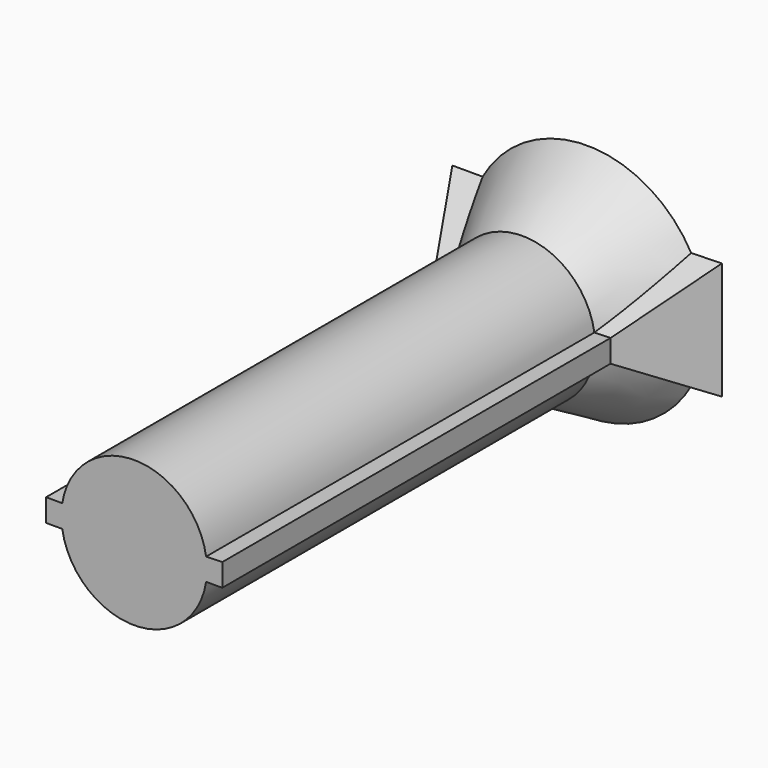
from build123d import *

# Parameters (mm, degrees)
F1_DEPTH               = 150
F2_DEPTH               = 25
DRAFT_F2_DRAFTED_ANGLE = -30


# Not quite as in the source:
# - an extrude with a draft is written as a straight extrude whose walls are then drafted


with BuildPart() as f1:
    # F0 (on Front) → F1 (new body)
    with BuildSketch(Plane.XZ):
        with BuildLine():
            ThreePointArc((22.2314160966, -3.4556680013), (22.4296056885, -1.7411981749), (22.4957987085, -0.0165810045))
            ThreePointArc((22.4957987085, -0.0165810045), (22.4300515903, 1.7022260351), (22.2331944739, 3.4109880427))
            ThreePointArc((22.2331944739, 3.4109880427), (0.0324511096, 22.4833891422), (-22.2303120623, 3.4834189955))
            ThreePointArc((-22.2303120623, 3.4834189955), (-22.5042012915, -0.0165810045), (-22.2303120623, -3.5165810045))
            ThreePointArc((-22.2303120623, -3.5165810045), (0.0266239001, -22.5165598891), (22.2314160966, -3.4556680013))
        make_face()
        with BuildLine():
            ThreePointArc((-22.2303120623, -3.5165810045), (-22.5042012915, -0.0165810045), (-22.2303120623, 3.4834189955))
            Line((-22.2303120623, 3.4834189955), (-27.2303120623, 3.4834189955))
            Line((-27.2303120623, 3.4834189955), (-27.2303120623, -3.5165810045))
            Line((-27.2303120623, -3.5165810045), (-22.2303120623, -3.5165810045))
        make_face()
        with BuildLine():
            ThreePointArc((22.2331944739, 3.4109880427), (22.4300515903, 1.7022260351), (22.4957987085, -0.0165810045))
            ThreePointArc((22.4957987085, -0.0165810045), (22.4296056885, -1.7411981749), (22.2314160966, -3.4556680013))
            Line((22.2314160966, -3.4556680013), (27.2314160966, -3.4556680013))
            Line((27.2314160966, -3.4556680013), (27.2314160966, 3.5443319987))
            Line((27.2314160966, 3.5443319987), (22.2331944739, 3.4109880427))
        make_face()
    extrude(amount=F1_DEPTH)


with BuildPart() as f2_drafted:
    # F2 (new): a face of the model
    f2_faces = [f1.part.faces().sort_by_distance(p)[0] for p in [
        (-0.0079243698, 0, -0.0160022595),
    ]]
    extrude(f2_faces, amount=F2_DEPTH)

    # draft_F2_drafted
    draft_f2_drafted_walls = [f2_drafted.faces().sort_by_distance(p)[0] for p in [
        (-24.7303120623, 16.6666666667, 3.4834189955),
        (-27.2303120623, 16.6666666667, -0.0165810045),
        (-24.7303120623, 16.6666666667, -3.5165810045),
        (0.0266239001, 16.6666666667, -22.5165598891),
        (24.7314160966, 16.6666666667, -3.4556680013),
        (27.2314160966, 16.6666666667, 0.0443319987),
        (24.7323052853, 16.6666666667, 3.4776600207),
        (0.0324511096, 16.6666666667, 22.4833891422),
    ]]
    draft(draft_f2_drafted_walls, neutral_plane=Plane(origin=(-0.0079243698, 0, -0.0160022595), x_dir=(1, 0, 0), z_dir=(0, 1, 0)), angle=DRAFT_F2_DRAFTED_ANGLE)


with BuildPart() as f1_1:
    add(f1.part)

    # join_F2_drafted: union F2_drafted
    add(f2_drafted.part)


solid = f1_1.part
